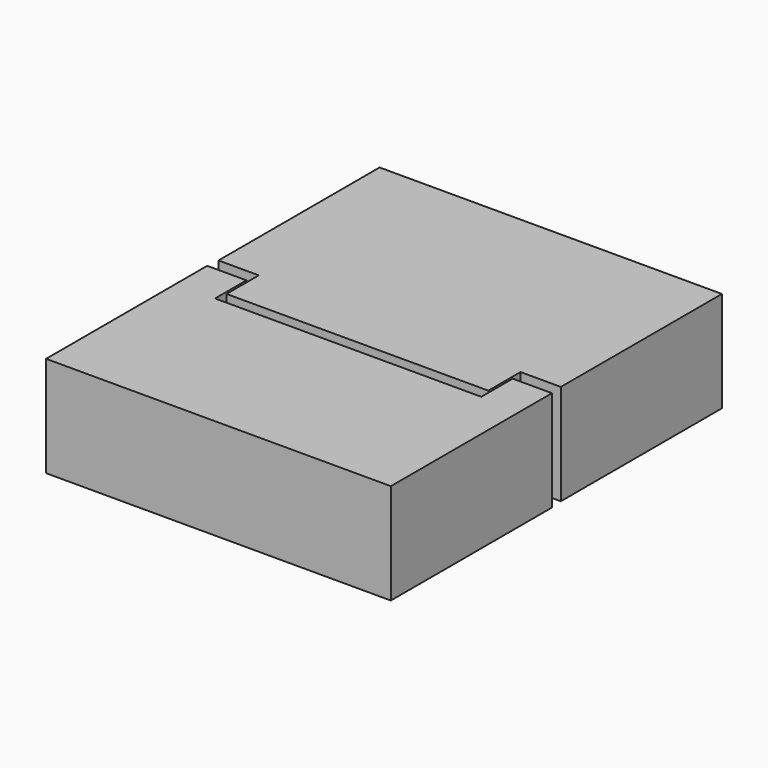
from build123d import *

# Parameters (mm, degrees)
F1_DEPTH = 10
F3_W     = 24.5
F3_H     = 19.5466473553
F4_DEPTH = 3
F5_W     = 24.5
F5_H     = 12.2730633011
F6_DEPTH = 3


with BuildPart() as f1:
    # F0 (on Top) → F1 (new body)
    with BuildSketch(Plane.XY):
        Polygon((-13, 0), (13, 0), (13, 4), (17, 4), (17, 24), (-17, 24), (-17, 4), (-13, 4), align=None)
    extrude(amount=F1_DEPTH)

    # F3 (on offset) → F4 (cut)
    with BuildSketch(Plane.XY.offset(5)):
        with Locations((0.0700059757, 9.7733236776)):
            Rectangle(F3_W, F3_H)
    extrude(amount=-F4_DEPTH, mode=Mode.SUBTRACT)


with BuildPart() as f1b:
    # F0 (on Top) → F1, piece 2 (new body)
    with BuildSketch(Plane.XY):
        Polygon((17.1204014808, 2.7489810166), (13.2204014808, 2.7489810166), (13.2204014808, -1.1510189834), (0, -1.1510189834), (-13.2204014808, -1.1510189834), (-13.2204014808, 2.7489810166), (-17.1204014808, 2.7489810166), (-17.1204014808, -17.2510189834), (17.1204014808, -17.2510189834), align=None)
    extrude(amount=F1_DEPTH)

    # F5 (on offset) → F6 (cut)
    with BuildSketch(Plane.XY.offset(5)):
        with Locations((0.0307181329, -7.0292878081)):
            Rectangle(F5_W, F5_H)
    extrude(amount=-F6_DEPTH, mode=Mode.SUBTRACT)


solid = Compound([f1.part, f1b.part])
